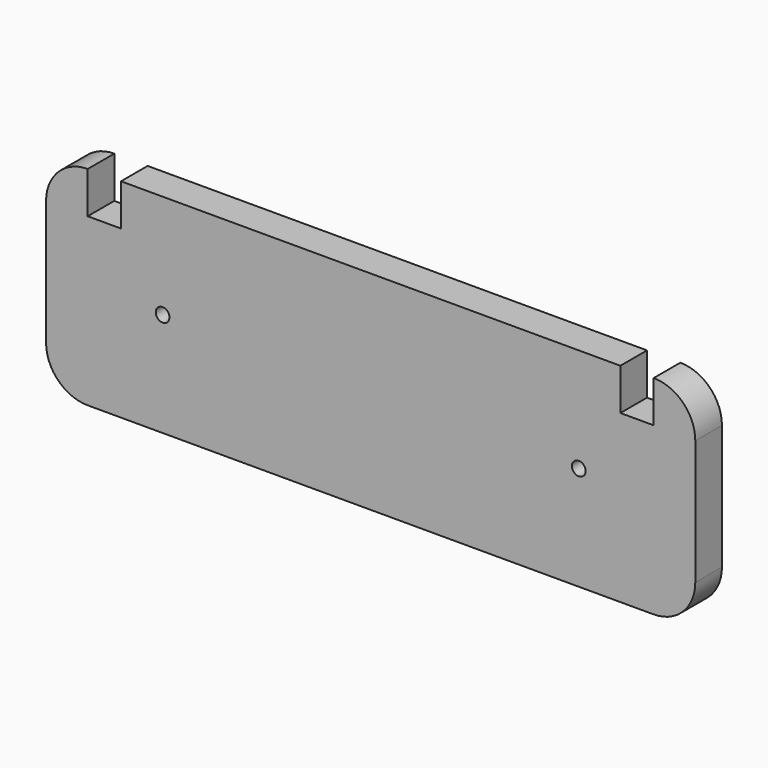
from build123d import *

# Parameters (mm, degrees)
F0_R     = 1.65
F1_DEPTH = 8
F2_R     = 9.99999


# Not quite as in the source:
# - a fillet or chamfer is up to 0.001 mm smaller than in the source, because OpenCascade refuses the exact size


with BuildPart() as f1:
    # F0 (on Front) → F1 (new body)
    with BuildSketch(Plane.XZ):
        Polygon((-27.0393844694, 188.5941594839), (92.9606155306, 188.5941594839), (110.9606155306, 188.5941594839), (110.9606155306, 238.5941594839), (100.9606155306, 238.5941594839), (100.9606155306, 228.5941594839), (92.9606155306, 228.5941594839), (92.9606155306, 238.5941594839), (-27.0393844694, 238.5941594839), (-27.0393844694, 228.5941594839), (-35.0393844694, 228.5941594839), (-35.0393844694, 238.5941594839), (-45.0393844694, 238.5941594839), (-45.0393844694, 188.5941594839), align=None)
        with Locations((-17.0393844694, 213.5941594839)):
            Circle(F0_R, mode=Mode.SUBTRACT)
        with Locations((82.9606155306, 213.5941594839)):
            Circle(F0_R, mode=Mode.SUBTRACT)
    extrude(amount=F1_DEPTH)

    # F2 (radius 10 in the source; OpenCascade refuses exactly that, so slightly less here)
    f2_edges = [f1.edges().sort_by_distance(p)[0] for p in [
        (-45.039384, -4, 238.594159),
        (-45.039384, -4, 188.594159),
        (110.960616, -4, 188.594159),
        (110.960616, -4, 238.594159),
    ]]
    fillet(f2_edges, radius=F2_R)


solid = f1.part
